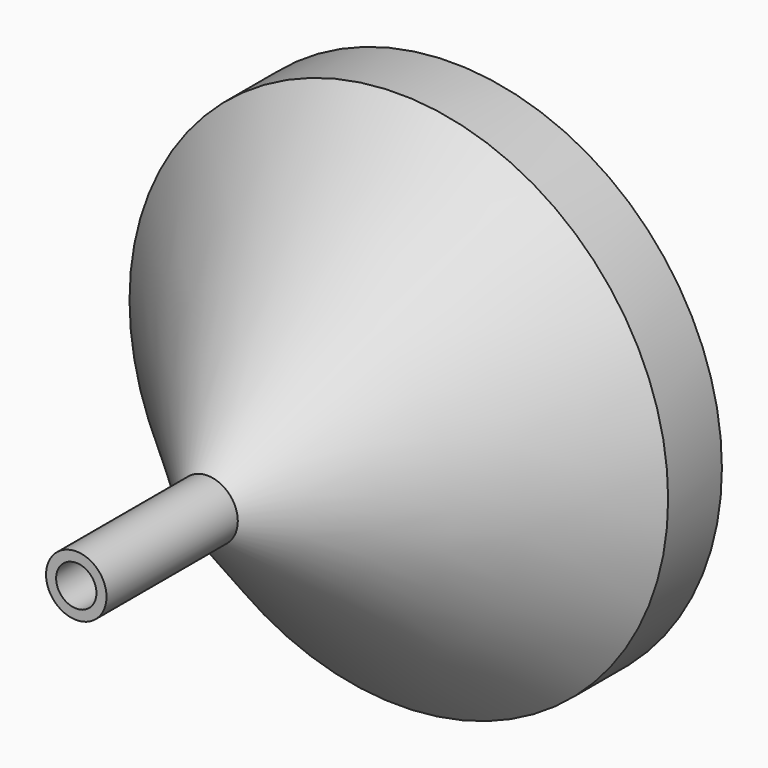
from build123d import *

# Parameters (mm, degrees)
F0_R     = 40.076976351
F0_R_2   = 4.5
F1_DEPTH = 50
F0_R_3   = 3
F3_DEPTH = 70
F4_SIZE  = 35


# Not quite as in the source:
# - a fillet or chamfer that OpenCascade refuses, or shapes differently, is made with other operations: its cross-section is extruded or revolved along the edge and cut away or added


with BuildPart() as f1:
    # F0 (on Front) → F1 (new body)
    with BuildSketch(Plane.XZ):
        Circle(F0_R)
        Circle(F0_R_2, mode=Mode.SUBTRACT)
    extrude(amount=F1_DEPTH)

    # F2: chamfer of 40 on 1 edges, made by hand

    # F2_s1 → F2_t2 (revolve, cut)
    with BuildSketch(Plane.XY):
        Polygon((40.076976351, -10), (0.076976351, -50), (40.076976351, -50), align=None)
    revolve(axis=Axis((0, -50, 0), (0, -1, 0)), mode=Mode.SUBTRACT)

    # F0 (on Front) → F3 (join)
    with BuildSketch(Plane.XZ):
        Circle(F0_R_2)
        Circle(F0_R_3, mode=Mode.SUBTRACT)
    extrude(amount=F3_DEPTH)

    # F4
    f4_edges = [f1.edges().sort_by_distance(p)[0] for p in [
        (-3, 0, 0),
    ]]
    chamfer(f4_edges, length=F4_SIZE)


solid = f1.part
